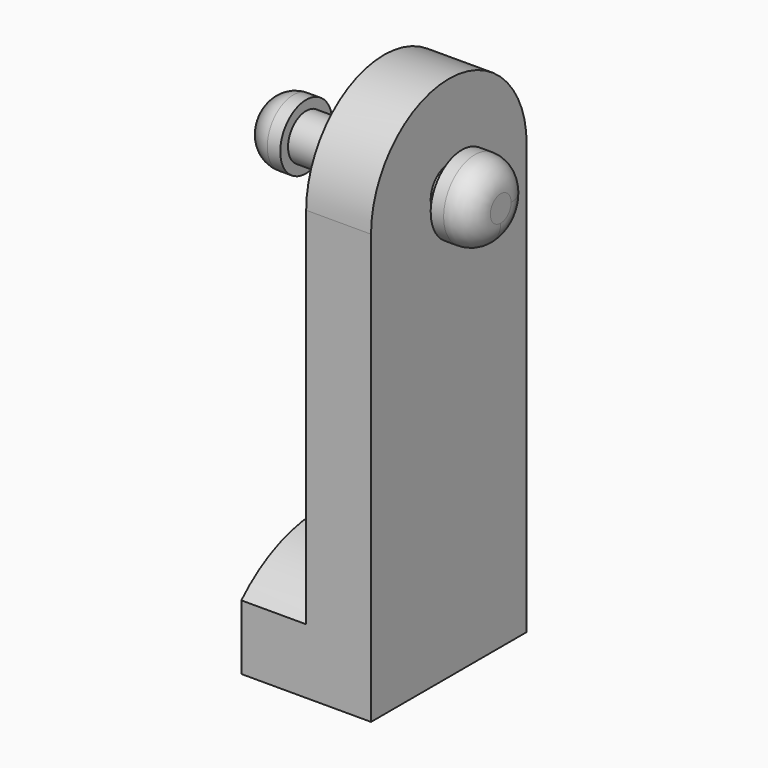
from build123d import *

# Parameters (mm, degrees)
F1_DEPTH = 5
F2_DEPTH = 5
F3_DEPTH = 6
F5_DEPTH = 3
F6_R     = 2
F7_DEPTH = 6
F8_R     = 2.5
F9_DEPTH = 3
F10_R    = 2


# Not quite as in the source:
# - a feature names something its author has since deleted; it is built from what else it names
# - the program builds the solid bodies; features that only make, move or delete a surface that nothing else refers to are left out


with BuildPart() as f1:
    # F0 (on Right) → F1 (new body)
    with BuildSketch(Plane.YZ):
        with BuildLine():
            ThreePointArc((7.5, 15), (0, 22.5), (-7.5, 15))
            Line((-7.5, 15), (-2, 15))
            ThreePointArc((-2, 15), (0, 17), (2, 15))
            Line((2, 15), (7.5, 15))
        make_face()
        with BuildLine():
            ThreePointArc((2, 15), (0, 17), (-2, 15))
            Line((-2, 15), (-1.95, 15))
            ThreePointArc((-1.95, 15), (0, 16.95), (1.95, 15))
            Line((1.95, 15), (2, 15))
        make_face()
        with BuildLine():
            ThreePointArc((1.95, 15), (0, 16.95), (-1.95, 15))
            Line((-1.95, 15), (-1.75, 15))
            ThreePointArc((-1.75, 15), (0, 16.75), (1.75, 15))
            Line((1.75, 15), (1.95, 15))
        make_face()
        with BuildLine():
            Line((-7.5, 15), (-7.5, -5.6289238692))
            ThreePointArc((-7.5, -5.6289238692), (0, -6.95), (7.5, -5.6289238692))
            Line((7.5, -5.6289238692), (7.5, 15))
            Line((7.5, 15), (2, 15))
            ThreePointArc((2, 15), (0, 13), (-2, 15))
            Line((-2, 15), (-7.5, 15))
        make_face()
        with BuildLine():
            Line((-1.95, 15), (-2, 15))
            ThreePointArc((-2, 15), (0, 13), (2, 15))
            Line((2, 15), (1.95, 15))
            ThreePointArc((1.95, 15), (0, 13.05), (-1.95, 15))
        make_face()
        with BuildLine():
            Line((-1.75, 15), (-1.95, 15))
            ThreePointArc((-1.95, 15), (0, 13.05), (1.95, 15))
            Line((1.95, 15), (1.75, 15))
            ThreePointArc((1.75, 15), (0, 13.25), (-1.75, 15))
        make_face()
        with BuildLine():
            Line((-7.5, -5.6289238692), (-7.5, -13.1065604925))
            ThreePointArc((-7.5, -13.1065604925), (0, -10), (7.5, -13.1065604925))
            Line((7.5, -13.1065604925), (7.5, -5.6289238692))
            ThreePointArc((7.5, -5.6289238692), (0, -6.95), (-7.5, -5.6289238692))
        make_face()
        with BuildLine():
            Line((-7.5, -13.1065604925), (-7.5, -18.1065604925))
            Line((-7.5, -18.1065604925), (7.5, -18.1065604925))
            Line((7.5, -18.1065604925), (7.5, -13.1065604925))
            ThreePointArc((7.5, -13.1065604925), (0, -10), (-7.5, -13.1065604925))
        make_face()
    extrude(amount=F1_DEPTH)

    # F0 (on Right) → F2 (join)
    with BuildSketch(Plane.YZ):
        with BuildLine():
            Line((-7.5, -13.1065604925), (-7.5, -18.1065604925))
            Line((-7.5, -18.1065604925), (7.5, -18.1065604925))
            Line((7.5, -18.1065604925), (7.5, -13.1065604925))
            ThreePointArc((7.5, -13.1065604925), (0, -10), (-7.5, -13.1065604925))
        make_face()
    extrude(amount=-F2_DEPTH)


with BuildPart() as f3:
    # F0 (on Right) → F3 (new body)
    with BuildSketch(Plane.YZ):
        with BuildLine():
            ThreePointArc((1.75, 15), (0, 16.75), (-1.75, 15))
            Line((-1.75, 15), (1.75, 15))
        make_face()
        with BuildLine():
            Line((1.75, 15), (-1.75, 15))
            ThreePointArc((-1.75, 15), (0, 13.25), (1.75, 15))
        make_face()
    extrude(amount=F3_DEPTH)

    # F4 (on face) → F5 (join)
    with BuildSketch(Plane.YZ.offset(6)):
        with BuildLine():
            ThreePointArc((0, 12), (2.1213203436, 12.8786796564), (3, 15))
            ThreePointArc((3, 15), (-2.1213203436, 17.1213203436), (0, 12))
        make_face()
    extrude(amount=F5_DEPTH)

    # F6
    f6_edges = [f3.edges().sort_by_distance(p)[0] for p in [
        (9, 0, 18),
    ]]
    fillet(f6_edges, radius=F6_R)


with BuildPart() as f7:
    # F0 (on Right) → F7 (new body)
    with BuildSketch(Plane.YZ):
        with BuildLine():
            ThreePointArc((1.75, 15), (0, 16.75), (-1.75, 15))
            Line((-1.75, 15), (1.75, 15))
        make_face()
        with BuildLine():
            Line((1.75, 15), (-1.75, 15))
            ThreePointArc((-1.75, 15), (0, 13.25), (1.75, 15))
        make_face()
    extrude(amount=-F7_DEPTH)

    # F8 (on face) → F9 (join)
    with BuildSketch(Plane(origin=(-6, 0, 0), x_dir=(0, -1, 0), z_dir=(-1, 0, 0))):
        with Locations((0, 15)):
            Circle(F8_R)
    extrude(amount=F9_DEPTH)

    # F10
    f10_edges = [f7.edges().sort_by_distance(p)[0] for p in [
        (-9, 2.5, 15),
    ]]
    fillet(f10_edges, radius=F10_R)


solid = Compound([f1.part, f3.part, f7.part])
